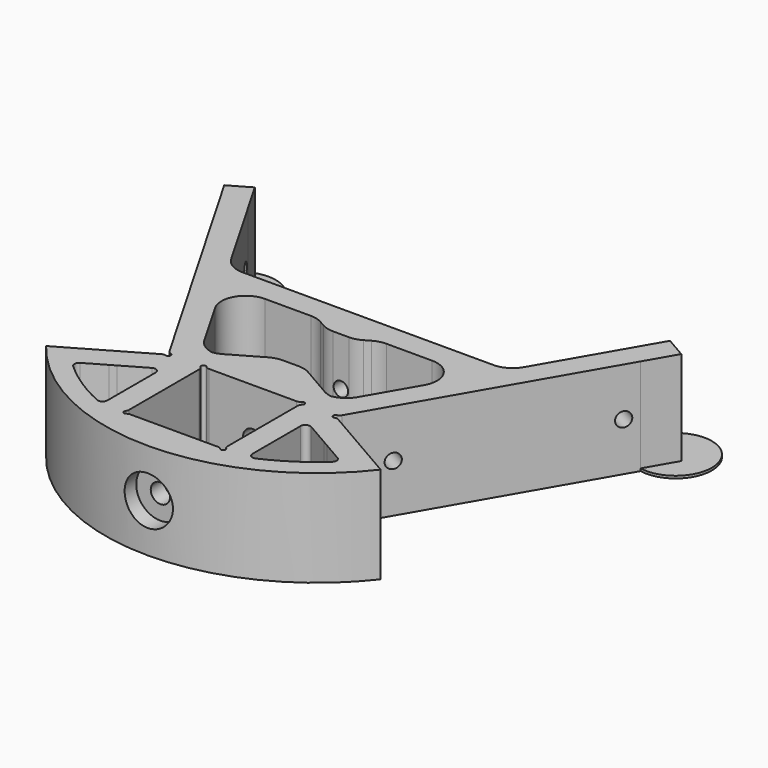
from build123d import *

# Parameters (mm, degrees)
F0_W            = 20.400000091
F0_H            = 20.400000091
F1_DEPTH        = 20
F7_D            = 3
F7_DEPTH        = 10
F7_TIP          = 0.9012909285
F8_D            = 3
F8_DEPTH        = 10
F8_TIP          = 0.9012909285
F9_D            = 3
F9_DEPTH        = 30
F9_TIP          = 0.9012909285
F10_D           = 4
F10_DEPTH       = 30
F10_START       = 0.3347373
F10_CBORE_D     = 10
F10_CBORE_DEPTH = 3
F10_TIP         = 1.2017212381
F11_D           = 1
F11_DEPTH       = 30
F11_TIP         = 0.3004303095
F12_R           = 1
F13_T1_DEPTH    = 20
F13_T3_DEPTH    = 26.6987298108
F14_DEPTH       = 0.5


# Not quite as in the source:
# - a fillet or chamfer that OpenCascade refuses, or shapes differently, is made with other operations: its cross-section is extruded or revolved along the edge and cut away or added


with BuildPart() as f1:
    # F0 (on Top) → F1 (new body)
    with BuildSketch(Plane.XY):
        Polygon((6.4641016151, 26.0483745358), (17.9807621135, 26.0483745358), (17.9807621135, 31.0483745358), (-17.9807621135, 31.0483745358), (-17.9807621135, 26.0483745358), (-6.4641016151, 26.0483745358), align=None)
        Polygon((-17.9807621135, 26.0483745358), (-17.9807621135, 31.0483745358), (-28.8675134595, 31.0483745358), (-25.9807621135, 26.0483745358), align=None)
        with BuildLine():
            Line((25.9807621135, 26.0483745358), (14.4337567297, 6.0483745358))
            Line((14.4337567297, 6.0483745358), (11.6602540378, 6.0483745358))
            Line((11.6602540378, 6.0483745358), (-11.6602540378, 6.0483745358))
            Line((-11.6602540378, 6.0483745358), (-14.4337567297, 6.0483745358))
            Line((-14.4337567297, 6.0483745358), (-25.9807621135, 26.0483745358))
            Line((-25.9807621135, 26.0483745358), (-28.8675134595, 31.0483745358))
            Line((-28.8675134595, 31.0483745358), (-39.4548471508, 49.3861744059))
            Line((-39.4548471508, 49.3861744059), (-42.9903810568, 55.5098987629))
            Line((-42.9903810568, 55.5098987629), (-47.3205080757, 53.0098987629))
            Line((-47.3205080757, 53.0098987629), (-43.7849741698, 46.8861744059))
            Line((-43.7849741698, 46.8861744059), (-17.3205080757, 1.0483745358))
            Line((-17.3205080757, 1.0483745358), (-34.6410161514, -8.9516254642))
            ThreePointArc((-34.6410161514, -8.9516254642), (0, -25.9516254642), (34.6410161514, -8.9516254642))
            Line((34.6410161514, -8.9516254642), (17.3205080757, 1.0483745358))
            Line((17.3205080757, 1.0483745358), (43.7849741698, 46.8861744059))
            Line((43.7849741698, 46.8861744059), (47.3205080757, 53.0098987629))
            Line((47.3205080757, 53.0098987629), (42.9903810568, 55.5098987629))
            Line((42.9903810568, 55.5098987629), (39.4548471508, 49.3861744059))
            Line((39.4548471508, 49.3861744059), (28.8675134595, 31.0483745358))
            Line((28.8675134595, 31.0483745358), (25.9807621135, 26.0483745358))
        make_face()
        with BuildLine():
            ThreePointArc((-22.7103164413, -14.9757110612), (-25.3474924854, -12.9844045429), (-27.8108891325, -10.7817524831))
            Line((-27.8108891325, -10.7817524831), (-22.5614149358, -7.7509671426))
            ThreePointArc((-22.5614149358, -7.7509671426), (-22.0073717449, -7.3757984906), (-21.4054445662, -7.0835673385))
            Line((-21.4054445662, -7.0835673385), (-15, -3.3853821939))
            Line((-15, -3.3853821939), (-15, -9.7067520427))
            Line((-15, -9.7067520427), (-15, -11.2055254497))
            ThreePointArc((-15, -11.2055254497), (-14.9961529432, -11.3149667107), (-14.9948703563, -11.424468055))
            ThreePointArc((-14.9948703563, -11.424468055), (-14.9961529432, -11.5339693994), (-15, -11.6434106603))
            Line((-15, -11.6434106603), (-15, -19.1411925583))
            ThreePointArc((-15, -19.1411925583), (-18.4907352427, -17.5253696018), (-21.8097023517, -15.5809998604))
            ThreePointArc((-21.8097023517, -15.5809998604), (-22.2776306814, -15.3045743127), (-22.7103164413, -14.9757110612))
        make_face(mode=Mode.SUBTRACT)
        with Locations((0, -8.9516254642)):
            Rectangle(F0_W, F0_H, mode=Mode.SUBTRACT)
        with BuildLine():
            Line((22.5667029919, -7.7540202032), (27.8108891325, -10.7817524831))
            ThreePointArc((27.8108891325, -10.7817524831), (25.350206463, -12.9821727678), (22.7160948799, -14.9717116082))
            ThreePointArc((22.7160948799, -14.9717116082), (22.280757774, -15.3029234672), (21.8097023517, -15.5809998604))
            ThreePointArc((21.8097023517, -15.5809998604), (18.4907352427, -17.5253696018), (15, -19.1411925583))
            Line((15, -19.1411925583), (15, -11.4242956019))
            Line((15, -11.4242956019), (15, -3.3853821939))
            Line((15, -3.3853821939), (21.4054445662, -7.0835673385))
            ThreePointArc((21.4054445662, -7.0835673385), (22.0102443295, -7.3769291493), (22.5667029919, -7.7540202032))
        make_face(mode=Mode.SUBTRACT)
        Polygon((-11.6602540378, 6.0483745358), (11.6602540378, 6.0483745358), (3, 11.0483745358), (-3, 11.0483745358), align=None)
        Polygon((3, 24.0483745358), (6.4641016151, 26.0483745358), (-6.4641016151, 26.0483745358), (-3, 24.0483745358), align=None)
        Polygon((17.9807621135, 26.0483745358), (25.9807621135, 26.0483745358), (28.8675134595, 31.0483745358), (17.9807621135, 31.0483745358), align=None)
        with BuildLine():
            ThreePointArc((21.8097023517, -15.5809998604), (22.280757774, -15.3029234672), (22.7160948799, -14.9717116082))
            ThreePointArc((22.7160948799, -14.9717116082), (22.2649828839, -15.2794563439), (21.8097023517, -15.5809998604))
        make_face()
        with BuildLine():
            ThreePointArc((-21.8097023517, -15.5809998604), (-22.2620666598, -15.2814164794), (-22.7103164413, -14.9757110612))
            ThreePointArc((-22.7103164413, -14.9757110612), (-22.2776306814, -15.3045743127), (-21.8097023517, -15.5809998604))
        make_face()
        with BuildLine():
            ThreePointArc((-21.4054445662, -7.0835673385), (-22.0073717449, -7.3757984906), (-22.5614149358, -7.7509671426))
            Line((-22.5614149358, -7.7509671426), (-21.4054445662, -7.0835673385))
        make_face()
        with BuildLine():
            Line((21.4054445662, -7.0835673385), (22.5667029919, -7.7540202032))
            ThreePointArc((22.5667029919, -7.7540202032), (22.0102443295, -7.3769291493), (21.4054445662, -7.0835673385))
        make_face()
    extrude(amount=F1_DEPTH)

    # F7
    with Locations(Plane(origin=(12.5364215664, -7.237906366, 0), x_dir=(0.5, 0.8660254038, 0), z_dir=(0.8660254038, -0.5, 0))):
        with Locations((19.5681730185, 10), (59.5681730185, 10)):
            Hole(F7_D / 2, depth=F7_DEPTH)
            with Locations((0, 0, -(F7_DEPTH + F7_TIP / 2))):  # 118° drill point
                Cone(0, F7_D / 2, F7_TIP, mode=Mode.SUBTRACT)

    # F8
    with Locations(Plane(origin=(-12.5364215664, -7.237906366, 0), x_dir=(0.5, -0.8660254038, 0), z_dir=(-0.8660254038, -0.5, 0))):
        with Locations((-19.5681730185, 10), (-59.5681730185, 10)):
            Hole(F8_D / 2, depth=F8_DEPTH)
            with Locations((0, 0, -(F8_DEPTH + F8_TIP / 2))):  # 118° drill point
                Cone(0, F8_D / 2, F8_TIP, mode=Mode.SUBTRACT)

    # F9
    with Locations(Plane(origin=(0, 31.0483745358, 0), x_dir=(-1, 0, 0), z_dir=(0, 1, 0))):
        with Locations((0, 10)):
            Hole(F9_D / 2, depth=F9_DEPTH)
            with Locations((0, 0, -(F9_DEPTH + F9_TIP / 2))):  # 118° drill point
                Cone(0, F9_D / 2, F9_TIP, mode=Mode.SUBTRACT)

    # F10
    # its depths count from where the whole tool has entered the part; down to there all is cleared
    with Locations(Plane.XZ.offset(26).offset(-F10_START)):
        with Locations((0, 10)):
            CounterBoreHole(F10_D / 2, F10_CBORE_D / 2, F10_CBORE_DEPTH, depth=F10_DEPTH)
            with Locations((0, 0, -(F10_DEPTH + F10_TIP / 2))):  # 118° drill point
                Cone(0, F10_D / 2, F10_TIP, mode=Mode.SUBTRACT)

    # F11
    with Locations(Plane(origin=(0, 0, 0), x_dir=(1, 0, 0), z_dir=(0, 0, -1))):
        with Locations((10.2000000455, -1.2483745813), (10.2000000455, 19.1516255097), (-10, 18.9516254642), (-10.2000000455, -1.2483745813), (-17.3205080757, -1.0483745358), (17.3205080757, -1.0483745358)):
            Hole(F11_D / 2, depth=F11_DEPTH)
            with Locations((0, 0, -(F11_DEPTH + F11_TIP / 2))):  # 118° drill point
                Cone(0, F11_D / 2, F11_TIP, mode=Mode.SUBTRACT)

    # F12
    f12_edges = [f1.edges().sort_by_distance(p)[0] for p in [
        (15, -19.141193, 10),
        (15, -3.385382, 10),
        (27.810889, -10.781752, 10),
        (-15, -3.385382, 10),
        (-27.810889, -10.781752, 10),
        (-15, -19.141193, 10),
        (-17.570508, 1.481387, 10),
        (17.570508, 1.481387, 10),
        (17.753521, 0.798375, 10),
        (-9.541742, -19.151626, 10),
        (9.7, -19.151626, 10),
        (10.2, -18.651626, 10),
        (10.2, 0.748375, 10),
        (9.7, 1.248375, 10),
        (-9.7, 1.248375, 10),
        (-10.2, 0.748375, 10),
        (-10.2, -18.493368, 10),
        (-17.753521, 0.798375, 10),
    ]]
    fillet(f12_edges, radius=F12_R)

    # F13: fillet of radius 5 on 14 edges, made by hand

    # F13_s2 → F13_t1 (join)
    with BuildSketch(Plane.XY):
        with BuildLine():
            ThreePointArc((-21.6506350946, 18.5483745358), (-21.6506350946, 23.5483745358), (-17.3205080757, 26.0483745358))
            Line((-17.3205080757, 26.0483745358), (-25.9807621135, 26.0483745358))
            Line((-25.9807621135, 26.0483745358), (-21.6506350946, 18.5483745358))
        make_face()
        with BuildLine():
            ThreePointArc((21.6506350946, 18.5483745358), (21.6506350946, 23.5483745358), (17.3205080757, 26.0483745358))
            Line((17.3205080757, 26.0483745358), (25.9807621135, 26.0483745358))
            Line((25.9807621135, 26.0483745358), (21.6506350946, 18.5483745358))
        make_face()
        with BuildLine():
            ThreePointArc((15.8771324027, 8.5483745358), (14.0470053838, 6.7182475169), (11.5470053838, 6.0483745358))
            Line((11.5470053838, 6.0483745358), (14.4337567297, 6.0483745358))
            Line((14.4337567297, 6.0483745358), (15.8771324027, 8.5483745358))
        make_face()
        with BuildLine():
            ThreePointArc((-11.5470053838, 6.0483745358), (-14.0470053838, 6.7182475169), (-15.8771324027, 8.5483745358))
            Line((-15.8771324027, 8.5483745358), (-14.4337567297, 6.0483745358))
            Line((-14.4337567297, 6.0483745358), (-11.5470053838, 6.0483745358))
        make_face()
        with BuildLine():
            ThreePointArc((-30.3108891325, 33.5483745358), (-28.4807621135, 31.7182475169), (-25.9807621135, 31.0483745358))
            Line((-25.9807621135, 31.0483745358), (-28.8675134595, 31.0483745358))
            Line((-28.8675134595, 31.0483745358), (-30.3108891325, 33.5483745358))
        make_face()
        with BuildLine():
            ThreePointArc((25.9807621135, 31.0483745358), (28.4807621135, 31.7182475169), (30.3108891325, 33.5483745358))
            Line((30.3108891325, 33.5483745358), (28.8675134595, 31.0483745358))
            Line((28.8675134595, 31.0483745358), (25.9807621135, 31.0483745358))
        make_face()
        with BuildLine():
            ThreePointArc((5.3038475773, 25.3785015547), (6.5097523518, 25.8780036673), (7.8038475773, 26.0483745358))
            Line((7.8038475773, 26.0483745358), (6.4641016151, 26.0483745358))
            Line((6.4641016151, 26.0483745358), (5.3038475773, 25.3785015547))
        make_face()
        with BuildLine():
            ThreePointArc((-7.8038475773, 26.0483745358), (-6.5097523518, 25.8780036673), (-5.3038475773, 25.3785015547))
            Line((-5.3038475773, 25.3785015547), (-6.4641016151, 26.0483745358))
            Line((-6.4641016151, 26.0483745358), (-7.8038475773, 26.0483745358))
        make_face()
        with BuildLine():
            ThreePointArc((-10.5, 6.7182475169), (-11.7059047745, 6.2187454044), (-13, 6.0483745358))
            Line((-13, 6.0483745358), (-11.6602540378, 6.0483745358))
            Line((-11.6602540378, 6.0483745358), (-10.5, 6.7182475169))
        make_face()
        with BuildLine():
            ThreePointArc((13, 6.0483745358), (11.7059047745, 6.2187454044), (10.5, 6.7182475169))
            Line((10.5, 6.7182475169), (11.6602540378, 6.0483745358))
            Line((11.6602540378, 6.0483745358), (13, 6.0483745358))
        make_face()
    extrude(amount=F13_T1_DEPTH)

    # F13_s4 → F13_t3 (cut)
    with BuildSketch(Plane.XY.offset(-3.3493649054)):
        with BuildLine():
            ThreePointArc((4.1602540378, 24.7182475169), (2.9543492634, 24.2187454044), (1.6602540378, 24.0483745358))
            Line((1.6602540378, 24.0483745358), (3, 24.0483745358))
            Line((3, 24.0483745358), (4.1602540378, 24.7182475169))
        make_face()
        with BuildLine():
            ThreePointArc((-1.6602540378, 24.0483745358), (-2.9543492634, 24.2187454044), (-4.1602540378, 24.7182475169))
            Line((-4.1602540378, 24.7182475169), (-3, 24.0483745358))
            Line((-3, 24.0483745358), (-1.6602540378, 24.0483745358))
        make_face()
        with BuildLine():
            ThreePointArc((-4.1602540378, 10.3785015547), (-2.9543492634, 10.8780036673), (-1.6602540378, 11.0483745358))
            Line((-1.6602540378, 11.0483745358), (-3, 11.0483745358))
            Line((-3, 11.0483745358), (-4.1602540378, 10.3785015547))
        make_face()
        with BuildLine():
            ThreePointArc((1.6602540378, 11.0483745358), (2.9543492634, 10.8780036673), (4.1602540378, 10.3785015547))
            Line((4.1602540378, 10.3785015547), (3, 11.0483745358))
            Line((3, 11.0483745358), (1.6602540378, 11.0483745358))
        make_face()
    extrude(amount=F13_T3_DEPTH, mode=Mode.SUBTRACT)

    # F0 (on Top) → F14 (join)
    with BuildSketch(Plane.XY):
        with BuildLine():
            Line((-42.9903810568, 55.5098987629), (-39.4548471508, 49.3861744059))
            ThreePointArc((-39.4548471508, 49.3861744059), (-48.9054445662, 60.7550892913), (-43.7849741698, 46.8861744059))
            Line((-43.7849741698, 46.8861744059), (-47.3205080757, 53.0098987629))
            Line((-47.3205080757, 53.0098987629), (-42.9903810568, 55.5098987629))
        make_face()
        with BuildLine():
            ThreePointArc((43.7849741698, 46.8861744059), (48.9054445662, 60.7550892913), (39.4548471508, 49.3861744059))
            Line((39.4548471508, 49.3861744059), (42.9903810568, 55.5098987629))
            Line((42.9903810568, 55.5098987629), (47.3205080757, 53.0098987629))
            Line((47.3205080757, 53.0098987629), (43.7849741698, 46.8861744059))
        make_face()
    extrude(amount=F14_DEPTH)


solid = f1.part
